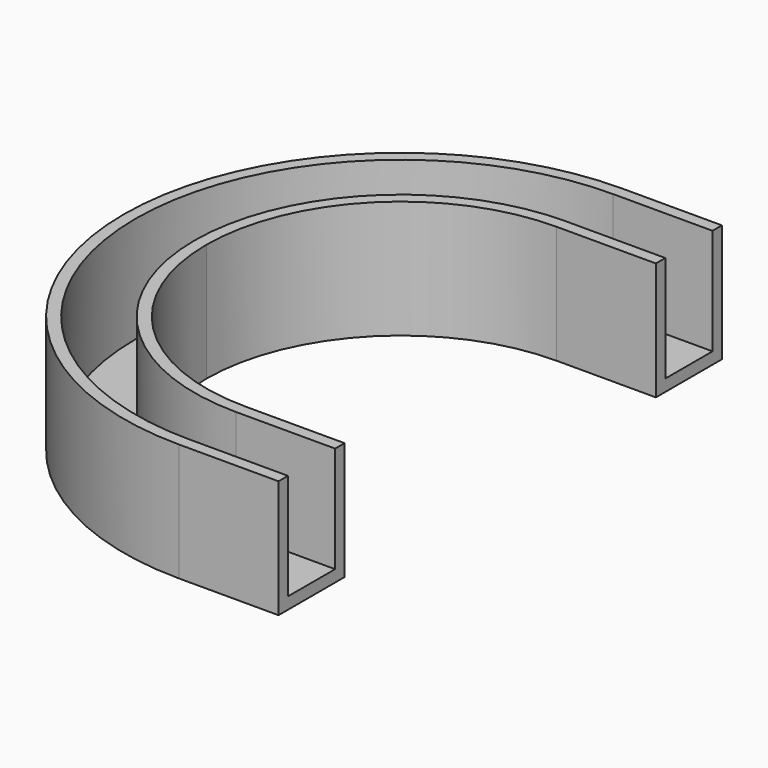
from build123d import *

# Parameters (mm, degrees)
F0_W     = 16.8362744153
F0_H     = 2
F1_DEPTH = 20
F0_H_2   = 10
F2_DEPTH = 2


with BuildPart() as f1:
    # F0 (on Top) → F1 (new body)
    with BuildSketch(Plane.XY):
        with BuildLine():
            Line((0, 33), (0, 35))
            ThreePointArc((0, 35), (-24.7487373415, 24.7487373415), (-35, 0))
            Line((-35, 0), (-33, 0))
            ThreePointArc((-33, 0), (-23.3345237792, 23.3345237792), (0, 33))
        make_face()
        with Locations((8.4181372076, 34)):
            Rectangle(F0_W, F0_H)
        with BuildLine():
            Line((-33, 0), (-35, 0))
            ThreePointArc((-35, 0), (-24.7487373415, -24.7487373415), (0, -35))
            Line((0, -35), (0, -33))
            ThreePointArc((0, -33), (-23.3345237792, -23.3345237792), (-33, 0))
        make_face()
        with Locations((8.4181372076, -34)):
            Rectangle(F0_W, F0_H)
    extrude(amount=F1_DEPTH)



with BuildPart() as f1b:
    # F0 (on Top) → F1, piece 2 (new body)
    with BuildSketch(Plane.XY):
        with BuildLine():
            ThreePointArc((-45, 0), (-31.8198051534, 31.8198051534), (0, 45))
            Line((0, 45), (0, 47))
            ThreePointArc((0, 47), (-33.2340187158, 33.2340187158), (-47, 0))
            Line((-47, 0), (-45, 0))
        make_face()
        with Locations((8.4181372076, 46)):
            Rectangle(F0_W, F0_H)
        with BuildLine():
            ThreePointArc((0, -45), (-31.8198051534, -31.8198051534), (-45, 0))
            Line((-45, 0), (-47, 0))
            ThreePointArc((-47, 0), (-33.2340187158, -33.2340187158), (0, -47))
            Line((0, -47), (0, -45))
        make_face()
        with Locations((8.4181372076, -46)):
            Rectangle(F0_W, F0_H)
    extrude(amount=F1_DEPTH)


with BuildPart() as f1_1:
    add(f1.part)

    add(f1b.part)  # F2 merges F1b
    # F0 (on Top) → F2 (join)
    with BuildSketch(Plane.XY):
        with BuildLine():
            ThreePointArc((0, -35), (-24.7487373415, -24.7487373415), (-35, 0))
            Line((-35, 0), (-45, 0))
            ThreePointArc((-45, 0), (-31.8198051534, -31.8198051534), (0, -45))
            Line((0, -45), (0, -35))
        make_face()
        with BuildLine():
            ThreePointArc((-35, 0), (-24.7487373415, 24.7487373415), (0, 35))
            Line((0, 35), (0, 45))
            ThreePointArc((0, 45), (-31.8198051534, 31.8198051534), (-45, 0))
            Line((-45, 0), (-35, 0))
        make_face()
        with Locations((8.4181372076, 40)):
            Rectangle(F0_W, F0_H_2)
        with Locations((8.4181372076, -40)):
            Rectangle(F0_W, F0_H_2)
    extrude(amount=F2_DEPTH)


solid = f1_1.part
